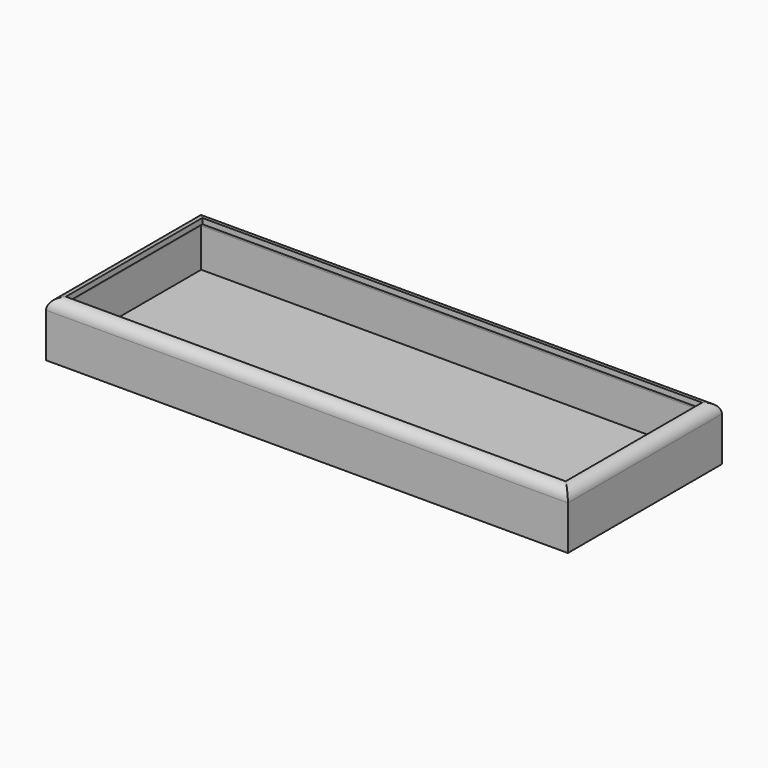
from build123d import *

# Parameters (mm, degrees)
F0_W     = 240.4982224107
F0_H     = 88.7339375913
F1_DEPTH = 25.4
F2_R     = 5.08
F3_T     = -2.54


# Not quite as in the source:
# - a shell that OpenCascade refuses in one call is made with other operations: the cavity is built on its own and cut out


with BuildPart() as f1:
    # F0 (on Top) → F1 (new body)
    with BuildSketch(Plane.XY):
        with Locations((-4.0379799902, 3.4744311124)):
            Rectangle(F0_W, F0_H)
    extrude(amount=F1_DEPTH)

    # F2
    f2_edges = [f1.edges().sort_by_distance(p)[0] for p in [
        (-4.03798, 47.8414, 25.4),
        (-124.287091, 3.474431, 25.4),
        (-4.03798, -40.892538, 25.4),
        (116.211131, 3.474431, 25.4),
    ]]
    fillet(f2_edges, radius=F2_R)

    # F3: a shell. OpenCascade refuses it in one call, so the cavity is built on its own and cut out:
    # the body offset inwards by the wall thickness, plus a prism from it out through each open face.
    f3_core = offset(f1.part, amount=F3_T, mode=Mode.PRIVATE)
    f3_exits = [f3_core.faces().sort_by_distance(p)[0] for p in [
        (-4.03798, 3.474431, 22.86),
    ]]
    add(f3_core, mode=Mode.SUBTRACT)
    extrude(f3_exits, amount=-F3_T, mode=Mode.SUBTRACT)


solid = f1.part
